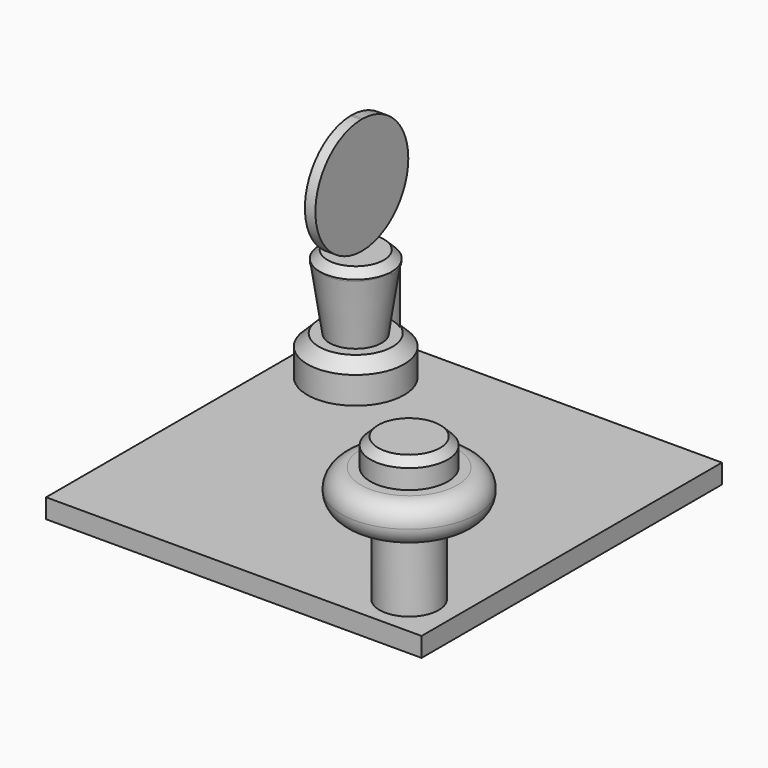
from build123d import *

# Parameters (mm, degrees)
F0_W      = 97
F0_H      = 5
F1_DEPTH  = 48.5
F2_R      = 7.6458649313
F3_DEPTH  = 20
F4_SIZE   = 2
F5_R      = 17.4861306414
F6_DEPTH  = 10
F7_R      = 4.99999
F8_R      = 10
F9_DEPTH  = 7
F10_SIZE  = 2
F11_R     = 12.5
F12_DEPTH = 10
F13_SIZE  = 3
F14_R     = 9.2774942081
F15_DEPTH = 19
F16_SIZE  = 2
F17_W     = 2.7091787755
F17_H     = 30.5535356402
F18_DEPTH = 30
F20_DEPTH = 17.3555893878


# Not quite as in the source:
# - a fillet or chamfer is up to 0.001 mm smaller than in the source, because OpenCascade refuses the exact size


with BuildPart() as f1:
    # F0 (on Front) → F1 (new body, symmetric)
    with BuildSketch(Plane.XZ):
        with Locations((1.2960880995, -0.2472623394)):
            Rectangle(F0_W, F0_H)
    extrude(amount=F1_DEPTH, both=True)

    # F2 (on face) → F3 (join)
    with BuildSketch(Plane.XY.offset(2.2527376606)):
        with Locations((37.7960880995, -37.5)):
            Circle(F2_R)
    extrude(amount=F3_DEPTH)

    # F4
    f4_edges = [f1.edges().sort_by_distance(p)[0] for p in [
        (30.150223, -37.5, 22.252738),
    ]]
    chamfer(f4_edges, length=F4_SIZE)

    # F5 (on face) → F6 (join)
    with BuildSketch(Plane.XY.offset(22.2527376606)):
        with Locations((37.7960880995, -37.5)):
            Circle(F5_R)
    extrude(amount=F6_DEPTH)

    # F7 (radius 5 in the source; OpenCascade refuses exactly that, so slightly less here)
    f7_edges = [f1.edges().sort_by_distance(p)[0] for p in [
        (55.282219, -37.5, 27.252738),
        (20.309957, -37.5, 22.252738),
        (20.309957, -37.5, 32.252738),
    ]]
    fillet(f7_edges, radius=F7_R)

    # F8 (on face) → F9 (join)
    with BuildSketch(Plane.XY.offset(32.2527376606)):
        with Locations((37.7960880995, -37.5)):
            Circle(F8_R)
    extrude(amount=F9_DEPTH)

    # F10
    f10_edges = [f1.edges().sort_by_distance(p)[0] for p in [
        (27.796088, -37.5, 39.252738),
    ]]
    chamfer(f10_edges, length=F10_SIZE)

    # F11 (on face) → F12 (join)
    with BuildSketch(Plane.XY.offset(2.2527376606)):
        with Locations((-31.2039119005, 31.5)):
            Circle(F11_R)
    extrude(amount=F12_DEPTH)

    # F13
    f13_edges = [f1.edges().sort_by_distance(p)[0] for p in [
        (-43.703912, 31.5, 12.252738),
    ]]
    chamfer(f13_edges, length=F13_SIZE)

    # F14 (on face) → F15 (join)
    with BuildSketch(Plane.XY.offset(12.2527376606)):
        with Locations((-31.2039119005, 31.5)):
            Circle(F14_R)
    extrude(amount=F15_DEPTH)

    # F16
    f16_edges = [f1.edges().sort_by_distance(p)[0] for p in [
        (-40.481406, 31.5, 31.252738),
    ]]
    chamfer(f16_edges, length=F16_SIZE)

    # F17 (on face) → F18 (join)
    with BuildSketch(Plane.XY.offset(31.2527376606)):
        with Locations((-31.2039119005, 31.5)):
            Rectangle(F17_W, F17_H)
    extrude(amount=F18_DEPTH)

    # F19 (on face) → F20 (cut, through all)
    with BuildSketch(Plane.YZ.offset(-29.8493225127)):
        with BuildLine():
            Line((46.7767678201, 61.2527376606), (32.0485214627, 61.2527376606))
            ThreePointArc((32.0485214627, 61.2527376606), (42.4791618872, 56.763699091), (46.7767678201, 46.2527376606))
            Line((46.7767678201, 46.2527376606), (46.7767678201, 61.2527376606))
        make_face()
        with BuildLine():
            ThreePointArc((31.5, 31.2527376606), (16.7717536426, 46.2527376606), (31.5, 61.2527376606))
            Line((31.5, 61.2527376606), (16.2232321799, 61.2527376606))
            Line((16.2232321799, 61.2527376606), (16.2232321799, 31.2527376606))
            Line((16.2232321799, 31.2527376606), (24.3496846545, 31.2527376606))
            Line((24.3496846545, 31.2527376606), (31.5, 31.2527376606))
        make_face()
        with BuildLine():
            ThreePointArc((46.7767678201, 46.2527376606), (42.4791618872, 35.7417762302), (32.0485214627, 31.2527376606))
            Line((32.0485214627, 31.2527376606), (38.6503153455, 31.2527376606))
            Line((38.6503153455, 31.2527376606), (46.7767678201, 31.2527376606))
            Line((46.7767678201, 31.2527376606), (46.7767678201, 46.2527376606))
        make_face()
    extrude(amount=-F20_DEPTH, mode=Mode.SUBTRACT)

    # F22 (on offset) → F23 (revolve, cut)
    with BuildSketch(Plane.XZ.offset(-31.4)):
        Polygon((-21.9264176924, 12.2527376606), (-21.9264176924, 29.2527376606), (-24.4411546737, 12.2527376606), align=None)
        Polygon((-37.9155091941, 12.2527376606), (-40.4814061086, 29.2527376606), (-40.4814061086, 12.2527376606), align=None)
    revolve(axis=Axis((-31.1523377895, 31.4, 20.637573155), (0, 0, 1)), mode=Mode.SUBTRACT)


solid = f1.part
